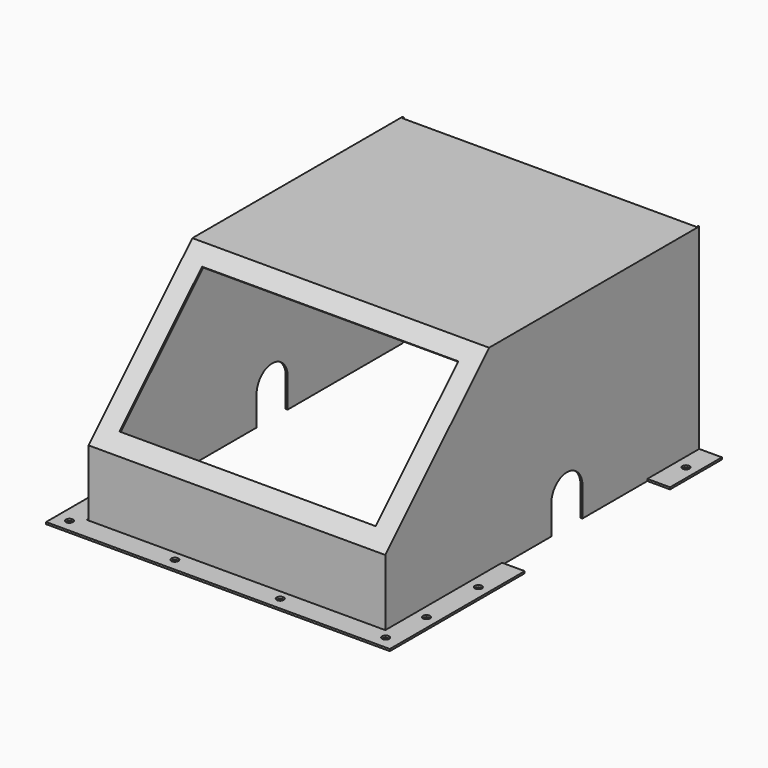
from build123d import *

# Parameters (mm, degrees)
F1_DEPTH  = 457.5
F2_T      = -6
F4_DEPTH  = 6
F5_R      = 11
F6_DEPTH  = 6
F5_W      = 70
F5_H      = 200
F8_DEPTH  = 985.001
F9_W      = 790
F9_H      = 450
F10_DEPTH = 6


with BuildPart() as f1:
    # F0 (on Right) → F1 (new body, symmetric)
    with BuildSketch(Plane.YZ):
        Polygon((-95.1616466045, 0), (1114.8383533955, 0), (1114.8383533955, 610), (304.8383533955, 610), (-95.1616466045, 210), align=None)
    extrude(amount=F1_DEPTH, both=True)

    # F2
    f2_openings = [f1.faces().sort_by_distance(p)[0] for p in [
        (0, 509.838353, 0),
    ]]
    offset(amount=F2_T, openings=f2_openings)

    # F3 (on face) → F4 (cut)
    with BuildSketch(Plane(origin=(0, 1114.8383533955, 0), x_dir=(-1, 0, 0), z_dir=(0, 1, 0))):
        Polygon((454, 0), (452.7580738068, 610), (-454, 610), (-454, 0), align=None)
    extrude(amount=-F4_DEPTH, mode=Mode.SUBTRACT)

    # F7 (on face) → F8 (cut, through all)
    with BuildSketch(Plane(origin=(-457.5, 0, 0), x_dir=(0, -1, 0), z_dir=(-1, 0, 0))):
        with BuildLine():
            Line((-664.8383533955, 90), (-664.8383533955, 0))
            Line((-664.8383533955, 0), (-544.8383533955, 0))
            Line((-544.8383533955, 0), (-544.8383533955, 90))
            ThreePointArc((-544.8383533955, 90), (-604.8383533955, 150), (-664.8383533955, 90))
        make_face()
    extrude(amount=-F8_DEPTH, mode=Mode.SUBTRACT)

    # F9 (on face) → F10 (cut)
    with BuildSketch(Plane(origin=(0, -152.5808233023, 152.5808233023), x_dir=(1, 0, 0), z_dir=(0, -0.7071067812, 0.7071067812))):
        with Locations((0, 364.3884033755)):
            Rectangle(F9_W, F9_H)
    extrude(amount=-F10_DEPTH, mode=Mode.SUBTRACT)


with BuildPart() as f6:
    # F5 (on face) → F6 (new body)
    with BuildSketch(Plane(origin=(0, 0, 0), x_dir=(1, 0, 0), z_dir=(0, 0, -1))):
        Polygon((-532.5, -354.8383533955), (-462.5, -354.8383533955), (-462.5, 95.1616466045), (457.5, 95.1616466045), (457.5, -354.8383533955), (527.5, -354.8383533955), (527.5, 165.1616466045), (-532.5, 165.1616466045), align=None)
        with Locations((-492.5, -219.8383533955)):
            Circle(F5_R, mode=Mode.SUBTRACT)
        with Locations((-492.5, -19.8383533955)):
            Circle(F5_R, mode=Mode.SUBTRACT)
        with Locations((-492.5, 125.1616466045)):
            Circle(F5_R, mode=Mode.SUBTRACT)
        with Locations((-167.5, 125.1616466045)):
            Circle(F5_R, mode=Mode.SUBTRACT)
        with Locations((492.5, -219.8383533955)):
            Circle(F5_R, mode=Mode.SUBTRACT)
        with Locations((157.5, 125.1616466045)):
            Circle(F5_R, mode=Mode.SUBTRACT)
        with Locations((492.5, -19.8383533955)):
            Circle(F5_R, mode=Mode.SUBTRACT)
        with Locations((482.5, 125.1616466045)):
            Circle(F5_R, mode=Mode.SUBTRACT)
    extrude(amount=-F6_DEPTH)


with BuildPart() as f6b:
    # F5 (on face) → F6, piece 2 (new body)
    with BuildSketch(Plane(origin=(0, 0, 0), x_dir=(1, 0, 0), z_dir=(0, 0, -1))):
        with Locations((-492.5, -1014.8383533955)):
            Rectangle(F5_W, F5_H)
        with Locations((-492.5, -1019.8383533955)):
            Circle(F5_R, mode=Mode.SUBTRACT)
    extrude(amount=-F6_DEPTH)


with BuildPart() as f6c:
    # F5 (on face) → F6, piece 3 (new body)
    with BuildSketch(Plane(origin=(0, 0, 0), x_dir=(1, 0, 0), z_dir=(0, 0, -1))):
        with Locations((492.5, -1014.8383533955)):
            Rectangle(F5_W, F5_H)
        with Locations((492.5, -1019.8383533955)):
            Circle(F5_R, mode=Mode.SUBTRACT)
    extrude(amount=-F6_DEPTH)


solid = Compound([f1.part, f6.part, f6b.part, f6c.part])
